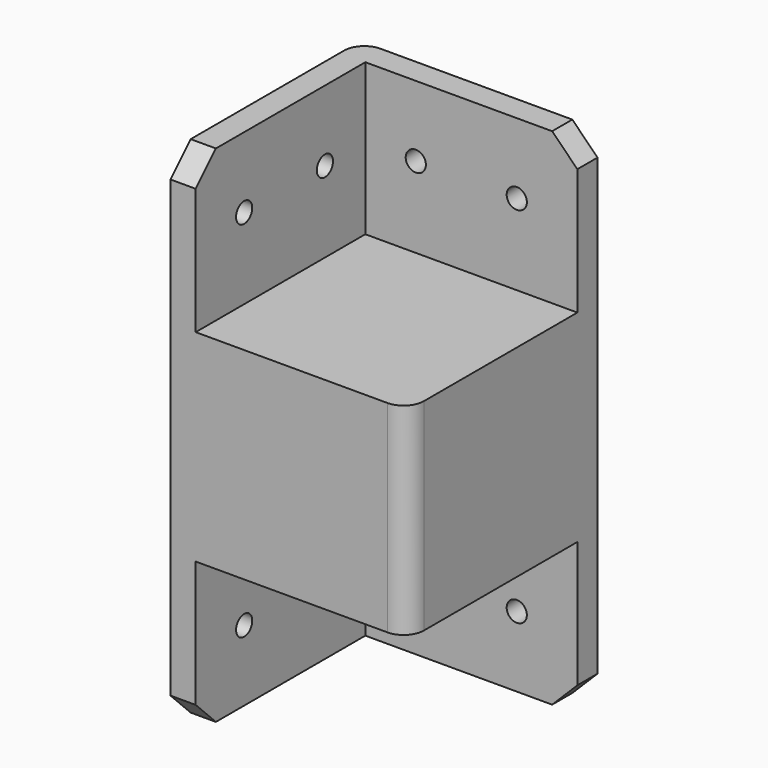
from build123d import *

# Parameters (mm, degrees)
F0_W          = 59.69
F0_H          = 59.69
F1_DEPTH      = 25.4
F1_DEPTH_BACK = 25.4
F3_DEPTH      = 38.1
F4_SIZE       = 6.35
F5_R          = 5.08
F6_R          = 5.08
F7_R          = 2.54
F8_DEPTH      = 25.4
F9_R          = 2.54
F10_DEPTH     = 25.4


# Not quite as in the source:
# - a pattern or mirror of a feature is missing from the dataset's text; its kind, count and spacing are read off the source's solid


with BuildPart() as f1:
    # F0 (on Top) → F1 (new body, two sides)
    with BuildSketch(Plane.XY) as f1_sk:
        Rectangle(F0_W, F0_H)
    extrude(amount=F1_DEPTH)
    extrude(f1_sk.sketch, amount=-F1_DEPTH_BACK)

    # F2 (on face) → F3 (join)
    with BuildSketch(Plane.XY.offset(25.4)):
        Polygon((-23.495, 23.495), (29.845, 23.495), (29.845, 29.845), (-29.845, 29.845), (-29.845, -29.845), (-23.495, -29.845), align=None)
    f3 = extrude(amount=F3_DEPTH)

    # F3_copies: F3 across plane
    add(f3.mirror(Plane(origin=(0, 0, 0), x_dir=(-1, 0, 0), z_dir=(0, 0, -1))))

    # F4
    f4_edges = [f1.edges().sort_by_distance(p)[0] for p in [
        (-26.67, -29.845, 63.5),
        (29.845, 26.67, 63.5),
        (-26.67, -29.845, -63.5),
        (29.845, 26.67, -63.5),
    ]]
    chamfer(f4_edges, length=F4_SIZE)

    # F5
    f5_edges = [f1.edges().sort_by_distance(p)[0] for p in [
        (29.845, -29.845, 0),
    ]]
    fillet(f5_edges, radius=F5_R)

    # F6
    f6_edges = [f1.edges().sort_by_distance(p)[0] for p in [
        (-29.845, 29.845, 0),
    ]]
    fillet(f6_edges, radius=F6_R)

    # F7 (on face) → F8 (cut)
    with BuildSketch(Plane.XZ.offset(-23.495)):
        with Locations((-10.795, 45.72)):
            Circle(F7_R)
        with Locations((14.605, 45.72)):
            Circle(F7_R)
    f8 = extrude(amount=-F8_DEPTH, mode=Mode.SUBTRACT)

    # F8_copies: F8 across plane
    add(f8.mirror(Plane(origin=(0, 0, 0), x_dir=(-1, 0, 0), z_dir=(0, 0, -1))), mode=Mode.SUBTRACT)

    # F9 (on face) → F10 (cut)
    with BuildSketch(Plane.YZ.offset(-23.495)):
        with Locations((-14.605, 45.72)):
            Circle(F9_R)
        with Locations((10.795, 45.72)):
            Circle(F9_R)
    f10 = extrude(amount=-F10_DEPTH, mode=Mode.SUBTRACT)

    # F10_copies: F10 across plane
    add(f10.mirror(Plane(origin=(0, 0, 0), x_dir=(-1, 0, 0), z_dir=(0, 0, -1))), mode=Mode.SUBTRACT)


solid = f1.part
